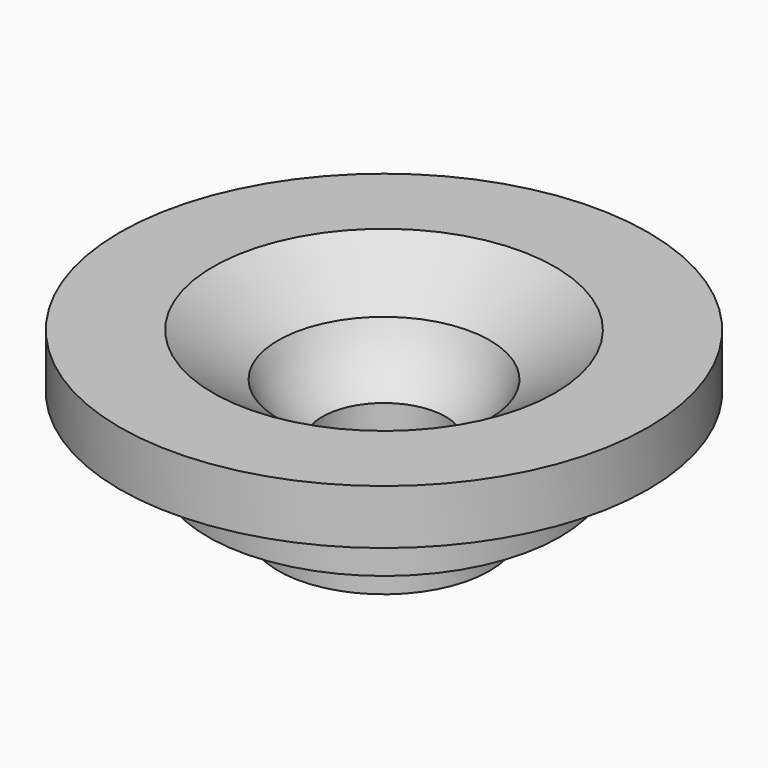
from build123d import *

# Parameters (mm, degrees)
F0_R     = 7.5
F0_R_2   = 1.75
F1_DEPTH = 5.05


# Not quite as in the source:
# - a fillet or chamfer that OpenCascade refuses, or shapes differently, is made with other operations: its cross-section is extruded or revolved along the edge and cut away or added


with BuildPart() as f1:
    # F0 (on Top) → F1 (new body)
    with BuildSketch(Plane.XY):
        Circle(F0_R)
        Circle(F0_R_2, mode=Mode.SUBTRACT)
    extrude(amount=F1_DEPTH)

    # F2 (on Front) → F3 (revolve, cut)
    with BuildSketch(Plane.XZ):
        Polygon((3, 1.5), (3, 0), (7.75, 0), (7.75, 3.5), (5, 3.5), (5, 1.5), align=None)
        with BuildLine():
            Line((0, 5.05), (0, 1.8))
            ThreePointArc((0, 1.8), (3.25, 5.05), (0, 8.3))
            Line((0, 8.3), (0, 5.05))
        make_face()
    revolve(axis=Axis((0, 0, 2.525), (0, 0, 1)), mode=Mode.SUBTRACT)

    # F4: chamfer of 2 on 1 edges, made by hand

    # F4_s1 → F4_t2 (revolve, cut)
    with BuildSketch(Plane.XZ):
        with BuildLine():
            Line((4.8541219597, 5.05), (3.0049326417, 3.8119047619))
            ThreePointArc((3.0049326417, 3.8119047619), (3.1823683685, 4.3904307714), (3.25, 5.05))
            Line((3.25, 5.05), (4.8541219597, 5.05))
        make_face()
    revolve(axis=Axis((0, 0, 5.05), (0, 0, 1)), mode=Mode.SUBTRACT)


solid = f1.part
